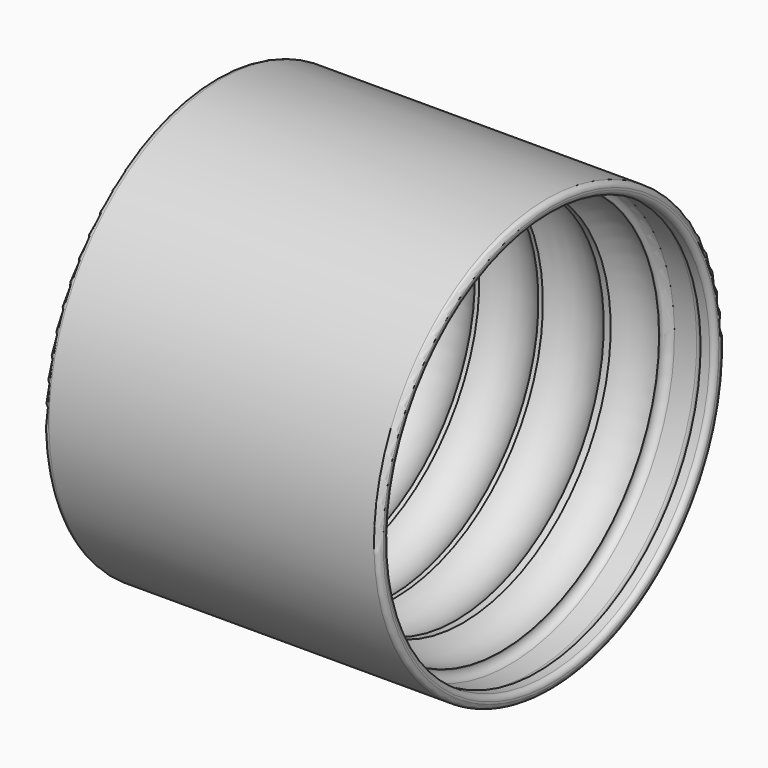
from build123d import *

# Parameters (mm, degrees)
F2_R = 0.5
F4_R = 1.25
F5_R = 1.5


# Not quite as in the source:
# - a fillet or chamfer that OpenCascade refuses, or shapes differently, is made with other operations: its cross-section is extruded or revolved along the edge and cut away or added


with BuildPart() as f1:
    # F0 (on Front) → F1 (revolve)
    with BuildSketch(Plane.XZ):
        with BuildLine():
            Line((82.5, 50), (82.5, 53))
            Line((82.5, 53), (0, 53))
            Line((0, 53), (0, 44))
            Line((0, 44), (5, 44))
            Line((5, 44), (5, 47.8))
            Line((5, 47.8), (10, 47.8))
            Line((10, 47.8), (10, 44))
            Line((10, 44), (11.4, 44))
            ThreePointArc((11.4, 44), (19.0365134749, 48.6643650208), (27.3484099858, 45.35))
            Line((27.3484099858, 45.35), (28.4484099858, 45.35))
            ThreePointArc((28.4484099858, 45.35), (35.6899882075, 48.7), (42.9315664293, 45.35))
            Line((42.9315664293, 45.35), (44.0315664293, 45.35))
            ThreePointArc((44.0315664293, 45.35), (51.5, 48.7), (58.9684335707, 45.35))
            Line((58.9684335707, 45.35), (60.6684335707, 45.35))
            ThreePointArc((60.6684335707, 45.35), (64.9158653321, 48.1670558963), (70, 48.5249038647))
            Line((70, 48.5249038647), (70, 50.75))
            Line((70, 50.75), (79, 50.75))
            Line((79, 50.75), (79, 50))
            Line((79, 50), (82.5, 50))
        make_face()
    revolve(axis=Axis((2.4749229779, 0, 0), (1, 0, 0)))

    # F2
    f2_edges = [f1.edges().sort_by_distance(p)[0] for p in [
        (5, 0, -47.8),
        (10, 0, -47.8),
    ]]
    fillet(f2_edges, radius=F2_R)

    # F3: fillet of radius 2 on 2 edges, made by hand

    # F3_s1 → F3_t2 (revolve)
    with BuildSketch(Plane.XZ):
        with BuildLine():
            ThreePointArc((72, 50.75), (70.5857864376, 50.1642135624), (70, 48.75))
            Line((70, 48.75), (70, 50.75))
            Line((70, 50.75), (72, 50.75))
        make_face()
    revolve(axis=Axis((70, 0, 0), (1, 0, 0)))

    # F3_s3 → F3_t4 (revolve)
    with BuildSketch(Plane.XZ):
        with BuildLine():
            ThreePointArc((79, 50), (78.3047759042, 50.5527756377), (77.4387505004, 50.75))
            Line((77.4387505004, 50.75), (79, 50.75))
            Line((79, 50.75), (79, 50))
        make_face()
    revolve(axis=Axis((79, 0, 0), (1, 0, 0)))

    # F4
    f4_edges = [f1.edges().sort_by_distance(p)[0] for p in [
        (82.5, 0, -53),
        (82.5, 0, -50),
    ]]
    fillet(f4_edges, radius=F4_R)

    # F5
    f5_edges = [f1.edges().sort_by_distance(p)[0] for p in [
        (0, 0, -53),
    ]]
    fillet(f5_edges, radius=F5_R)


solid = f1.part
